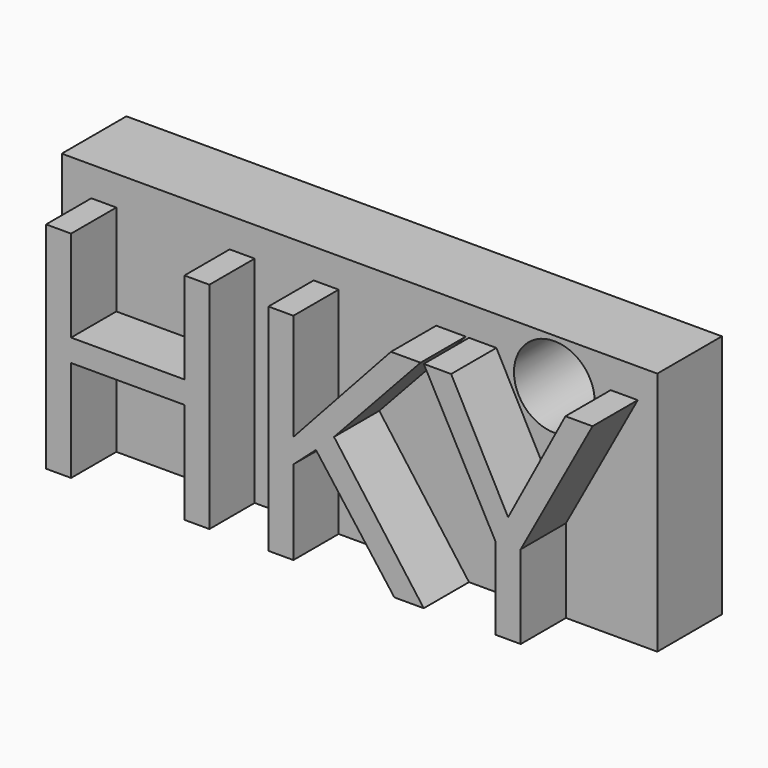
from build123d import *

# Parameters (mm, degrees)
F0_W         = 73.7206041813
F0_H         = 30.3053557873
F1_DEPTH     = 10
F2_TEXT_SIZE = 37.3003294142
F3_DEPTH     = 7
F5_D         = 10


# Not quite as in the source:
# - Text() gives the source's letters only with a copy of the font that has no kerning and outlines rounded to 1/6400 em; it was checked with that copy


with BuildPart() as f1:
    # F0 (on Front) → F1 (new body)
    with BuildSketch(Plane.XZ):
        with Locations((36.8603020906, 15.1526778936)):
            Rectangle(F0_W, F0_H)
    extrude(amount=F1_DEPTH)

    # F2 (on face) → F3 (join)
    with BuildSketch(Plane.XZ.offset(10)):
        with Locations((0, 0)):
            Text('HKY', F2_TEXT_SIZE, font='Open Sans', text_align=(TextAlign.LEFT, TextAlign.BOTTOM))
    extrude(amount=F3_DEPTH)

    # F5 (through all)
    with Locations(Plane.XZ.offset(10)):
        with Locations((60.9807744622, 24.7075520456)):
            Hole(F5_D / 2)


solid = f1.part
